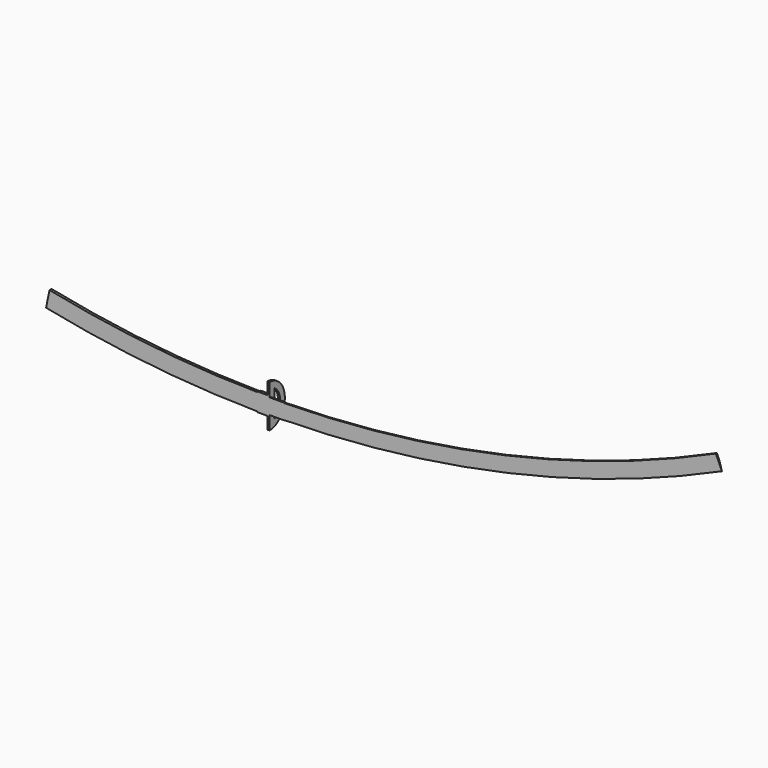
from build123d import *

# Parameters (mm, degrees)
F7_DEPTH = 0.3175


# Not quite as in the source:
# - ends of sketch curves that miss each other by under 0.0002 mm in the source are joined


with BuildPart() as f2:
    # F2: sweep along a path in F0
    with BuildLine(Plane.XZ) as f2_path:
        ThreePointArc((0, 0), (68.7773667676, 7.3040471778), (134.4866231347, 28.8903602567))
    # F1 (on Right) → F2 (sweep)
    with BuildSketch(Plane.YZ):
        Polygon((0, 1.905), (0, 0), (0, -2.54), (0.381, 0), (0.381, 1.905), align=None)
    sweep(path=f2_path.line)

    # F5: sweep along a path in F4
    with BuildLine(Plane.XZ) as f5_path:
        ThreePointArc((0, 0), (2.4458425758, 0.0091340961), (4.8915487069, 0.0365358747))
    # F3 (on Right) → F5 (sweep)
    with BuildSketch(Plane.YZ):
        Polygon((0, 2.032), (0, 0), (0, -2.6136133212), (0.1228220883, -2.5678527446), (0.508, 0), (0.508, 1.9473483553), align=None)
    sweep(path=f5_path.line)

    # F6 (on Right) → F7 (join, symmetric)
    with BuildSketch(Plane.YZ):
        with BuildLine():
            Line((0, 6.0325), (0, 0))
            Line((0, 0), (0, -0.3175))
            Line((0, -0.3175), (0, -6.6675))
            add(Edge.make_bspline(
                [(0, -6.6675), (5.715, -6.6675), (5.715, -0.3175), (5.715, 6.0325), (0, 6.0325)],
                knots=[0, 0, 0, 1.5707963268, 1.5707963268, 3.1415926536, 3.1415926536, 3.1415926536], degree=2, weights=[1, 0.7071067812, 1, 0.7071067812, 1]))
        make_face()
        with BuildLine():
            add(Edge.make_bspline(
                [(1.7779333577, -4.3936777564), (1.8932057262, -4.3256133179), (2.226963855, -4.1042878788), (2.7353351732, -3.6411355791), (3.2476945886, -2.9503867428), (3.6393859021, -2.1373354473), (3.8812326613, -1.2519774786), (3.9648836694, -0.3175), (3.8812326613, 0.6169774786), (3.6393859021, 1.5023354473), (3.2476945886, 2.3153867428), (2.7353351732, 3.0061355791), (2.2269638551, 3.4692878788), (1.8932057263, 3.6906133178), (1.7779333579, 3.7586777563)],
                knots=[0.0777545272, 0.0777545272, 0.0777545272, 0.0777545272, 0.09375, 0.125, 0.15625, 0.1875, 0.21875, 0.25, 0.28125, 0.3125, 0.34375, 0.375, 0.40625, 0.4222454727, 0.4222454727, 0.4222454727, 0.4222454727], degree=3))
            Line((1.7779333577, -4.3936777564), (1.7779333579, 3.7586777563))
        make_face(mode=Mode.SUBTRACT)
    extrude(amount=F7_DEPTH, both=True)

    # F9: sweep along a path in F0
    with BuildLine(Plane.XZ) as f9_path:
        ThreePointArc((0, 0), (-33.1178347786, 1.6789606381), (-65.896072187, 6.6986261303))
    # F8 (on Right) → F9 (sweep)
    with BuildSketch(Plane.YZ):
        with BuildLine():
            Line((0, 2.2225), (0, 0))
            Line((0, 0), (0, -0.3175))
            Line((0, -0.3175), (0, -2.8575))
            Line((0, -2.8575), (0.508, -2.8575))
            ThreePointArc((0.508, -2.8575), (1.0468153673, -2.6343153673), (1.27, -2.0955))
            Line((1.27, -2.0955), (1.27, 1.4605))
            ThreePointArc((1.27, 1.4605), (1.0468153673, 1.9993153673), (0.508, 2.2225))
            Line((0.508, 2.2225), (0, 2.2225))
        make_face()
    sweep(path=f9_path.line)

    # F12: sweep along a path in F11
    with BuildLine(Plane.XZ) as f12_path:
        ThreePointArc((0, 0), (-1.653886477, 0.0041766699), (-3.3077307637, 0.0167065731))
    # F10 (on Right) → F12 (sweep)
    with BuildSketch(Plane.YZ):
        Polygon((0, 2.413), (0, 0), (0, -3.048), (1.242357539, -2.760580508), (1.5768870944, -0.3175), (1.242357539, 2.125580508), align=None)
    sweep(path=f12_path.line)


solid = f2.part
